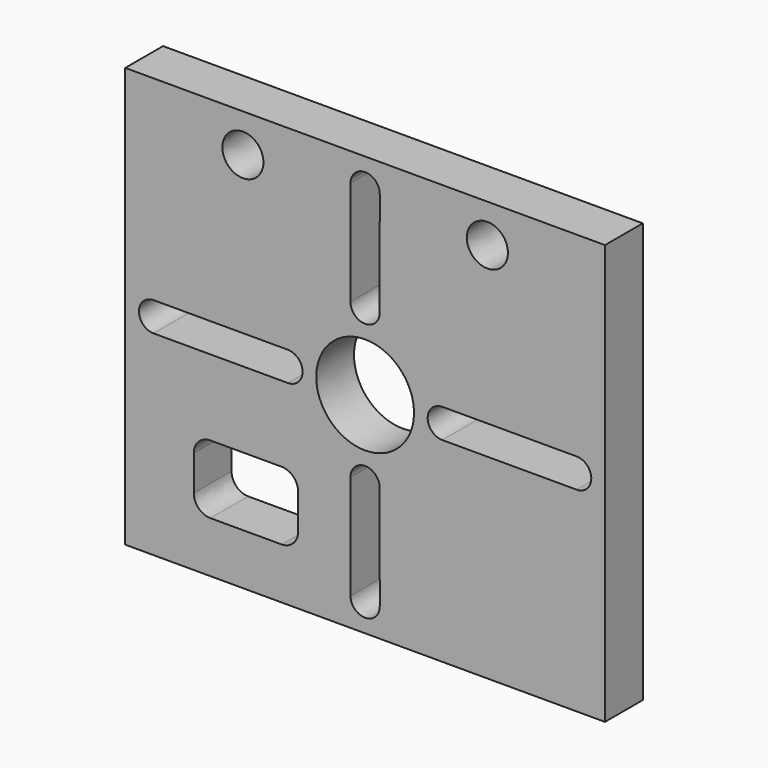
from build123d import *

# Parameters (mm, degrees)
F0_W     = 50.800353
F0_H     = 44.45
F1_DEPTH = 5


# Not quite as in the source:
# - ends of sketch curves that miss each other by under 0.0002 mm in the source are joined


with BuildPart() as f1:
    # F0 (on Front) → F1 (new body)
    with BuildSketch(Plane.XZ):
        with Locations((5e-07, 0)):
            Rectangle(F0_W, F0_H)
        with BuildLine():
            add(Edge.make_bspline(
                [(-7.08854, -11.336161), (-7.08854, -10.361789), (-7.878409, -9.572272), (-8.852429, -9.572272)],
                knots=[0, 0, 0, 0, 1, 1, 1, 1], degree=3))
            Line((-7.08854, -11.336161), (-7.08854, -15.052322))
            add(Edge.make_bspline(
                [(-8.852429, -16.816211), (-7.878409, -16.816211), (-7.08854, -16.026695), (-7.08854, -15.052322)],
                knots=[0, 0, 0, 0, 1, 1, 1, 1], degree=3))
            Line((-8.852429, -16.816211), (-16.378237, -16.816211))
            add(Edge.make_bspline(
                [(-18.142126, -15.052322), (-18.142126, -16.026695), (-17.352257, -16.816211), (-16.378237, -16.816211)],
                knots=[0, 0, 0, 0, 1, 1, 1, 1], degree=3))
            Line((-18.142126, -15.052322), (-18.142126, -11.336161))
            add(Edge.make_bspline(
                [(-16.378237, -9.572272), (-17.352257, -9.572272), (-18.142126, -10.361789), (-18.142126, -11.336161)],
                knots=[0, 0, 0, 0, 1, 1, 1, 1], degree=3))
            Line((-16.378237, -9.572272), (-8.852429, -9.572272))
        make_face(mode=Mode.SUBTRACT)
        with BuildLine():
            Line((-1.5500305536, -19.2250000002), (-1.5500305536, -8.1871465892))
            ThreePointArc((-1.5500305536, -8.1871465892), (-1.5500734508, -8.1804888446), (-1.55008775, -8.1738309772))
            ThreePointArc((-1.55008775, -8.1738309772), (-9.17611e-05, -6.6238309772), (1.54991225, -8.173822955))
            Line((1.54991225, -8.173822955), (1.5499694464, -19.224991978))
            ThreePointArc((1.5499694464, -19.224991978), (-2.65425e-05, -20.7749959891), (-1.5500305536, -19.2250000002))
        make_face(mode=Mode.SUBTRACT)
        with BuildLine():
            add(Edge.make_bspline(
                [(-0.0001188036, 5.1738309774), (-2.8576188036, 5.1738309774), (-5.1743108036, 2.8571389774), (-5.1743108036, -8.0226e-06)],
                knots=[0, 0, 0, 0, 1, 1, 1, 1], degree=3))
            add(Edge.make_bspline(
                [(5.1737201964, -8.0226e-06), (5.1737201964, 2.8571389774), (2.8573811964, 5.1738309774), (-0.0001188036, 5.1738309774)],
                knots=[0, 0, 0, 0, 1, 1, 1, 1], degree=3))
            add(Edge.make_bspline(
                [(-0.0001188036, -5.1742000226), (2.8573811964, -5.1742000226), (5.1737201964, -2.8578610226), (5.1737201964, -8.0226e-06)],
                knots=[0, 0, 0, 0, 1, 1, 1, 1], degree=3))
            add(Edge.make_bspline(
                [(-5.1743108036, -8.0226e-06), (-5.1743108036, -2.8578610226), (-2.8576188036, -5.1742000226), (-0.0001188036, -5.1742000226)],
                knots=[0, 0, 0, 0, 1, 1, 1, 1], degree=3))
        make_face(mode=Mode.SUBTRACT)
        with BuildLine():
            Line((-22.400176, 1.55), (-8.1743108036, 1.55))
            ThreePointArc((-8.1743108036, 1.55), (-6.624368, 0), (-8.174368, -1.55))
            Line((-8.174368, -1.55), (-22.400176, -1.55))
            ThreePointArc((-22.400176, -1.55), (-23.950176, 0), (-22.400176, 1.55))
        make_face(mode=Mode.SUBTRACT)
        with BuildLine():
            add(Edge.make_bspline(
                [(-12.941829, 20.343636), (-14.143743, 20.343636), (-15.117409, 19.369616), (-15.117409, 18.168055)],
                knots=[0, 0, 0, 0, 1, 1, 1, 1], degree=3))
            add(Edge.make_bspline(
                [(-10.766601, 18.168055), (-10.766601, 19.369616), (-11.740621, 20.343636), (-12.941829, 20.343636)],
                knots=[0, 0, 0, 0, 1, 1, 1, 1], degree=3))
            add(Edge.make_bspline(
                [(-12.941829, 15.992828), (-11.740621, 15.992828), (-10.766601, 16.966847), (-10.766601, 18.168055)],
                knots=[0, 0, 0, 0, 1, 1, 1, 1], degree=3))
            add(Edge.make_bspline(
                [(-15.117409, 18.168055), (-15.117409, 16.966847), (-14.143743, 15.992828), (-12.941829, 15.992828)],
                knots=[0, 0, 0, 0, 1, 1, 1, 1], degree=3))
        make_face(mode=Mode.SUBTRACT)
        with BuildLine():
            Line((-1.5500305536, 8.1871465892), (-1.5500305536, 19.2250000002))
            ThreePointArc((-1.5500305536, 19.2250000002), (-2.65425e-05, 20.7749959891), (1.5499694464, 19.224991978))
            Line((1.5499694464, 19.224991978), (1.54991225, 8.1738309772))
            ThreePointArc((1.54991225, 8.1738309772), (-9.17611e-05, 6.6238309772), (-1.55008775, 8.1738309772))
            Line((-1.55008775, 8.1738309772), (-1.5500305536, 8.1871465892))
        make_face(mode=Mode.SUBTRACT)
        with BuildLine():
            Line((8.1743108036, 1.55), (22.400176, 1.55))
            ThreePointArc((22.400176, 1.55), (23.950176, 0), (22.400176, -1.55))
            Line((22.400176, -1.55), (8.1743108036, -1.55))
            ThreePointArc((8.1743108036, -1.55), (6.624368, 0), (8.1743108036, 1.55))
        make_face(mode=Mode.SUBTRACT)
        with BuildLine():
            add(Edge.make_bspline(
                [(12.94571, 20.343636), (11.743796, 20.343636), (10.770129, 19.369616), (10.770129, 18.168055)],
                knots=[0, 0, 0, 0, 1, 1, 1, 1], degree=3))
            add(Edge.make_bspline(
                [(15.121291, 18.168055), (15.121291, 19.369616), (14.146918, 20.343636), (12.94571, 20.343636)],
                knots=[0, 0, 0, 0, 1, 1, 1, 1], degree=3))
            add(Edge.make_bspline(
                [(12.94571, 15.992828), (14.146918, 15.992828), (15.121291, 16.966847), (15.121291, 18.168055)],
                knots=[0, 0, 0, 0, 1, 1, 1, 1], degree=3))
            add(Edge.make_bspline(
                [(10.770129, 18.168055), (10.770129, 16.966847), (11.743796, 15.992828), (12.94571, 15.992828)],
                knots=[0, 0, 0, 0, 1, 1, 1, 1], degree=3))
        make_face(mode=Mode.SUBTRACT)
    extrude(amount=F1_DEPTH)


solid = f1.part
